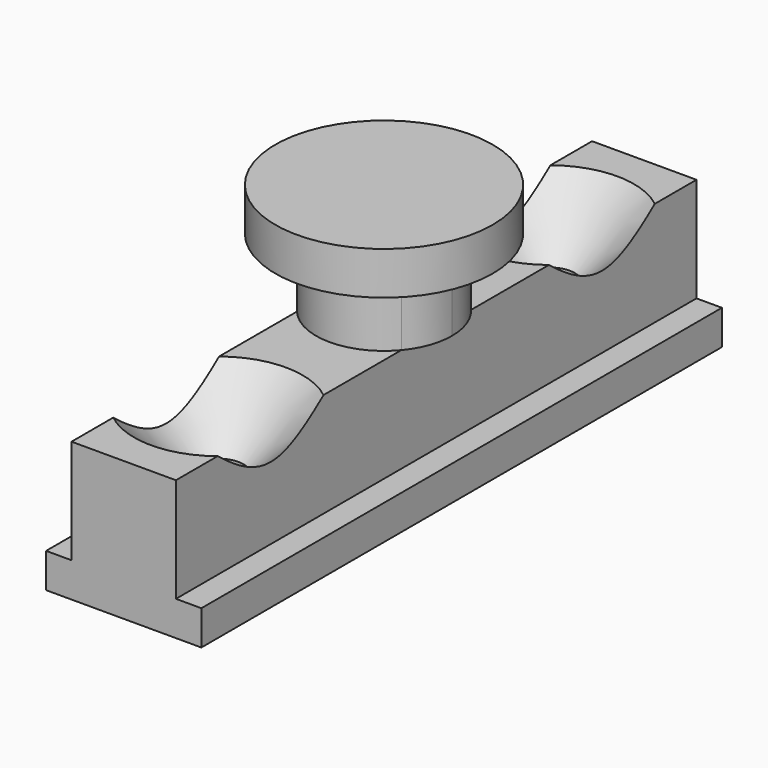
from build123d import *

# Parameters (mm, degrees)
F1_DEPTH = 22
F3_DEPTH = 2.3
F4_R     = 3.675
F4_R_2   = 2.3
F5_DEPTH = 1.45
F6_R     = 0.85
F7_DEPTH = 25


# Not quite as in the source:
# - a fillet or chamfer that OpenCascade refuses, or shapes differently, is made with other operations: its cross-section is extruded or revolved along the edge and cut away or added


with BuildPart() as f1:
    # F0 (on Front) → F1 (new body)
    with BuildSketch(Plane.XZ):
        Polygon((-36.1197131506, 22.3681449045), (-39.6497131506, 22.3681449045), (-39.6497131506, 18.8381449045), (-40.5097131506, 18.8381449045), (-40.5097131506, 17.6681449045), (-39.6497131506, 17.6681449045), (-36.1197131506, 17.6681449045), (-35.2597131506, 17.6681449045), (-35.2597131506, 18.8381449045), (-36.1197131506, 18.8381449045), align=None)
    extrude(amount=F1_DEPTH)

    # F2 (on face) → F3 (join)
    with BuildSketch(Plane.XY.offset(22.3681449045)):
        with BuildLine():
            Line((-36.1197131506, -12.4747118363), (-36.1197131506, -9.5252881637))
            ThreePointArc((-36.1197131506, -9.5252881637), (-37.8847131506, -8.7), (-39.6497131506, -9.5252881637))
            Line((-39.6497131506, -9.5252881637), (-39.6497131506, -12.4747118363))
            ThreePointArc((-39.6497131506, -12.4747118363), (-37.8847131506, -13.3), (-36.1197131506, -12.4747118363))
        make_face()
        with BuildLine():
            Line((-39.6497131506, -12.4747118363), (-39.6497131506, -9.5252881637))
            ThreePointArc((-39.6497131506, -9.5252881637), (-40.1847131506, -11), (-39.6497131506, -12.4747118363))
        make_face()
        with BuildLine():
            ThreePointArc((-36.1197131506, -12.4747118363), (-35.7225961325, -11.7843787351), (-35.5847131506, -11))
            ThreePointArc((-35.5847131506, -11), (-35.7225961325, -10.2156212649), (-36.1197131506, -9.5252881637))
            Line((-36.1197131506, -9.5252881637), (-36.1197131506, -12.4747118363))
        make_face()
    extrude(amount=F3_DEPTH)

    # F4 (on face) → F5 (join)
    with BuildSketch(Plane.XY.offset(24.6681449045)):
        with Locations((-37.8847131506, -11)):
            Circle(F4_R)
        with Locations((-37.8847131506, -11)):
            Circle(F4_R_2, mode=Mode.SUBTRACT)
        with Locations((-37.8847131506, -11)):
            Circle(F4_R_2)
    extrude(amount=F5_DEPTH)

    # F6 (on face) → F7 (cut)
    with BuildSketch(Plane(origin=(0, 0, 17.6681449045), x_dir=(1, 0, 0), z_dir=(0, 0, -1))):
        with Locations((-37.8847131506, 18)):
            Circle(F6_R)
        with Locations((-37.8847131506, 4)):
            Circle(F6_R)
    extrude(amount=-F7_DEPTH, mode=Mode.SUBTRACT)

    # F8: chamfer of 2 on 1 edges, made by hand

    # F8_s1 → F8_t2 (revolve, cut)
    with BuildSketch(Plane.XZ.offset(18)):
        Polygon((-35.0347131506, 22.3681449045), (-37.0347131506, 20.3681449045), (-37.0347131506, 22.3681449045), align=None)
    revolve(axis=Axis((-37.8847131506, -18, 22.3681449045), (0, 0, -1)), mode=Mode.SUBTRACT)

    # F9: chamfer of 2 on 1 edges, made by hand

    # F9_s1 → F9_t2 (revolve, cut)
    with BuildSketch(Plane.XZ.offset(4)):
        Polygon((-35.0347131506, 22.3681449045), (-37.0347131506, 20.3681449045), (-37.0347131506, 22.3681449045), align=None)
    revolve(axis=Axis((-37.8847131506, -4, 22.3681449045), (0, 0, -1)), mode=Mode.SUBTRACT)


solid = f1.part
